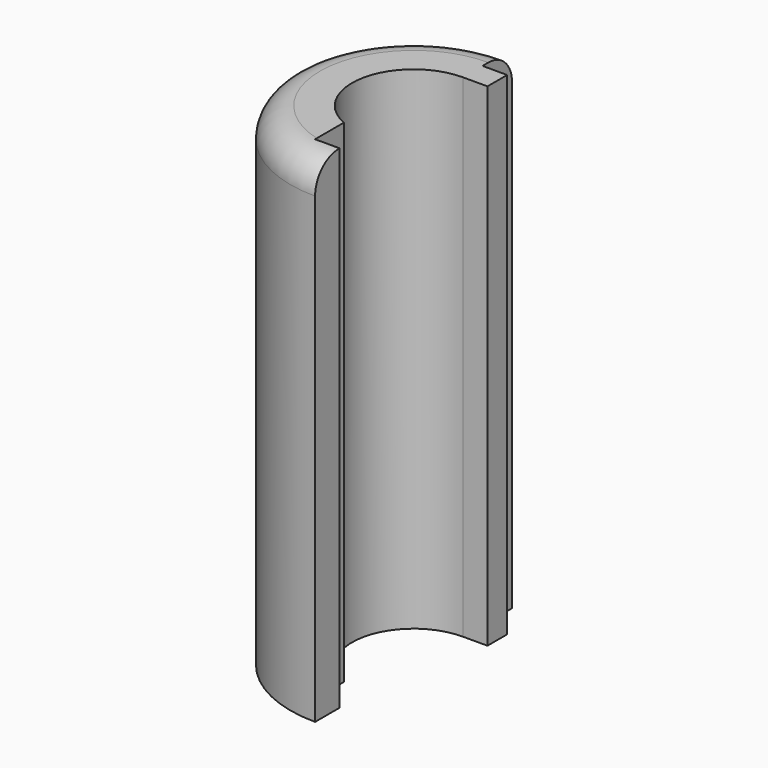
from build123d import *

# Parameters (mm, degrees)
F1_DEPTH    = 100
F2_T2_ANGLE = 248.8655063523


# Not quite as in the source:
# - a fillet or chamfer that OpenCascade refuses, or shapes differently, is made with other operations: its cross-section is extruded or revolved along the edge and cut away or added


with BuildPart() as f1:
    # F0 (on Top) → F1 (new body)
    with BuildSketch(Plane.XY):
        with BuildLine():
            ThreePointArc((-5, -11.4564392374), (-12.2363289116, 2.5538705461), (0, 12.5))
            Line((0, 12.5), (5, 12.5))
            Line((5, 12.5), (5, 17.5))
            Line((5, 17.5), (0, 17.5))
            Line((0, 17.5), (0, 25))
            ThreePointArc((0, 25), (-25, 0), (0, -25))
            Line((0, -25), (0, -18.75))
            Line((0, -18.75), (-5, -18.75))
            Line((-5, -18.75), (-5, -11.4564392374))
        make_face()
    extrude(amount=F1_DEPTH)

    # F2: fillet of radius 6 on 1 edges, made by hand

    # F2_s1 → F2_t2 (revolve, cut)
    with BuildSketch(Plane(origin=(0, 0, 0), x_dir=(0, 0, 1), z_dir=(0.8247903997, -0.5654385878, 0))):
        with BuildLine():
            ThreePointArc((94, -25), (98.2426406871, -23.2426406871), (100, -19))
            Line((100, -19), (100, -25))
            Line((100, -25), (94, -25))
        make_face()
    revolve(axis=Axis((0, 0, 100), (0, 0, 1)), revolution_arc=F2_T2_ANGLE, mode=Mode.SUBTRACT)


solid = f1.part
